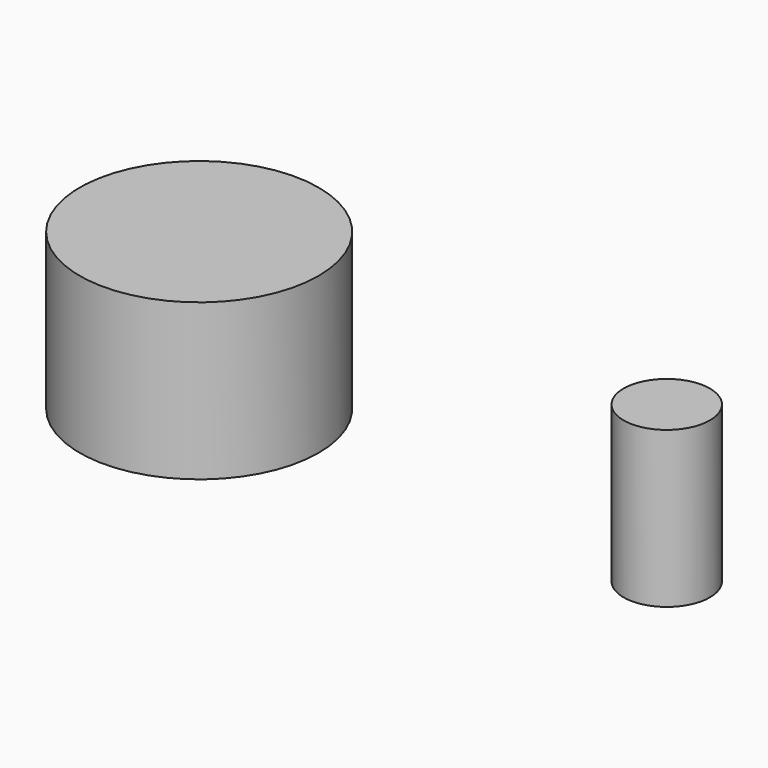
from build123d import *

# Parameters (mm, degrees)
F1_R     = 19.4796450826
F2_DEPTH = 25.4
F1_R_2   = 7.0338305057


# Not quite as in the source:
# - a feature names something its author has since deleted; it is built from what else it names


with BuildPart() as f2:
    # F1 (on Top) → F2 (new body)
    with BuildSketch(Plane.XY):
        with Locations((0, -50.8)):
            Circle(F1_R)
    extrude(amount=F2_DEPTH)


with BuildPart() as f2b:
    # F1 (on Top) → F2, piece 2 (new body)
    with BuildSketch(Plane.XY):
        with Locations((76.2, -50.8)):
            Circle(F1_R_2)
    extrude(amount=F2_DEPTH)


solid = Compound([f2.part, f2b.part])
